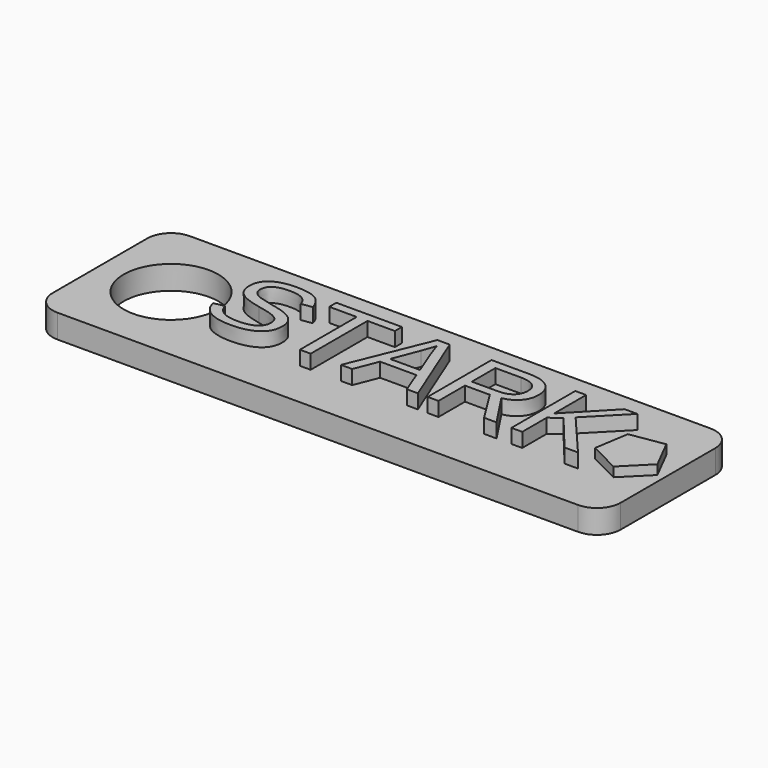
from build123d import *

# Parameters (mm, degrees)
F1_W         = 120
F1_H         = 35
F1_R         = 10
F2_DEPTH     = 5
F3_R         = 5
F0_TEXT_SIZE = 24.5115240496
F4_DEPTH     = 8
F6_DEPTH     = 7


# Not quite as in the source:
# - Text() gives the source's letters only with a copy of the font that has no kerning and outlines rounded to 1/6400 em; it was checked with that copy


with BuildPart() as f2:
    # F1 (on Top) → F2 (new body)
    with BuildSketch(Plane.XY):
        Rectangle(F1_W, F1_H)
        with Locations((-45, 0)):
            Circle(F1_R, mode=Mode.SUBTRACT)
    extrude(amount=F2_DEPTH)

    # F3
    f3_edges = [f2.edges().sort_by_distance(p)[0] for p in [
        (60, 17.5, 2.5),
        (60, -17.5, 2.5),
        (-60, 17.5, 2.5),
        (-60, -17.5, 2.5),
    ]]
    fillet(f3_edges, radius=F3_R)

    # F0 (on Top) → F4 (join)
    with BuildSketch(Plane.XY):
        with Locations((-34.5815494657, -7.3489006146)):
            Text('STARK', F0_TEXT_SIZE, font='Arimo', text_align=(TextAlign.LEFT, TextAlign.BOTTOM))
    extrude(amount=F4_DEPTH)

    # F5 (on Top) → F6 (join)
    with BuildSketch(Plane.XY):
        Polygon((53.3728079425, -6.1337688842), (58.5350839867, -0.9714945316), (55.2207003521, 5.5333522438), (48.0100225699, 4.3912942899), (46.8679622532, -2.819383118), align=None)
    extrude(amount=F6_DEPTH)


solid = f2.part
